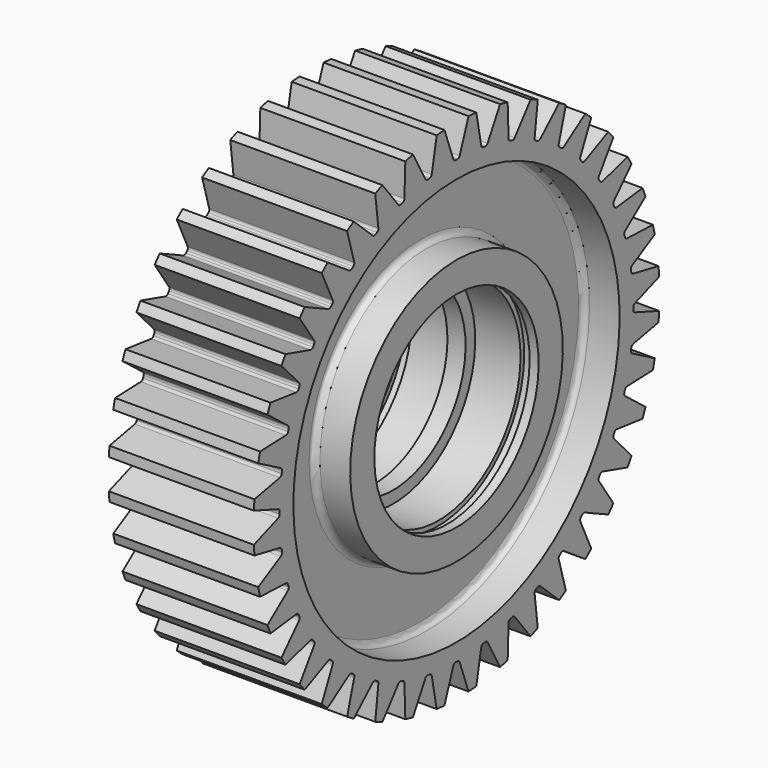
from build123d import *

# Parameters (mm, degrees)
F3_DEPTH        = 50
F3_COPIES_COUNT = 40


# Not quite as in the source:
# - a feature of the source that left no trace in its solid (it failed there, or was rolled back) is left out
# - a pattern or mirror of a feature is missing from the dataset's text; its kind, count and spacing are read off the source's solid


with BuildPart() as f1:
    # F0 (on Front) → F1 (revolve)
    with BuildSketch(Plane.XZ):
        with BuildLine():
            Line((0, 84), (-24, 84))
            Line((-24, 84), (-24, 67.5))
            Line((-24, 67.5), (-14, 67.5))
            ThreePointArc((-14, 67.5), (-12.5857864376, 66.9142135624), (-12, 65.5))
            Line((-12, 65.5), (-12, 46))
            ThreePointArc((-12, 46), (-12.5857864376, 44.5857864376), (-14, 44))
            Line((-14, 44), (-24, 44))
            Line((-24, 44), (-24, 34))
            Line((-24, 34), (-21, 34))
            Line((-21, 34), (-21, 35.5))
            Line((-21, 35.5), (-18, 35.5))
            Line((-18, 35.5), (-18, 34))
            Line((-18, 34), (-3, 34))
            Line((-3, 34), (-3, 30))
            Line((-3, 30), (0, 30))
            Line((0, 30), (3, 30))
            Line((3, 30), (3, 34))
            Line((3, 34), (18, 34))
            Line((18, 34), (18, 35.5))
            Line((18, 35.5), (21, 35.5))
            Line((21, 35.5), (21, 34))
            Line((21, 34), (24, 34))
            Line((24, 34), (24, 44))
            Line((24, 44), (14, 44))
            ThreePointArc((14, 44), (12.5857864376, 44.5857864376), (12, 46))
            Line((12, 46), (12, 65.5))
            ThreePointArc((12, 65.5), (12.5857864376, 66.9142135624), (14, 67.5))
            Line((14, 67.5), (24, 67.5))
            Line((24, 67.5), (24, 84))
            Line((24, 84), (0, 84))
        make_face()
    revolve(axis=Axis((-12, 0, 0), (1, 0, 0)))

    # F2 (on face) → F3 (cut)
    with BuildSketch(Plane.YZ.offset(24)):
        with BuildLine():
            ThreePointArc((0.385598978, 73.1530399645), (0.9591754143, 73.3338879202), (1.3252915988, 73.8110198211))
            Line((1.3252915988, 73.8110198211), (4.98, 83.8522486282))
            ThreePointArc((4.98, 83.8522486282), (0, 84), (-4.98, 83.8522486282))
            Line((-4.98, 83.8522486282), (-1.3252915988, 73.8110198211))
            ThreePointArc((-1.3252915988, 73.8110198211), (-0.9591754143, 73.3338879202), (-0.385598978, 73.1530399645))
            Line((-0.385598978, 73.1530399645), (0.385598978, 73.1530399645))
        make_face()
    f3 = extrude(amount=-F3_DEPTH, mode=Mode.SUBTRACT)

    # F3_copies: F3 ×40 about axis
    f3_copies_axis = Axis((0, 0, 0), (1, 0, 0))
    for i in range(1, F3_COPIES_COUNT):
        add(f3.rotate(f3_copies_axis, i * 360 / F3_COPIES_COUNT), mode=Mode.SUBTRACT)


solid = f1.part
